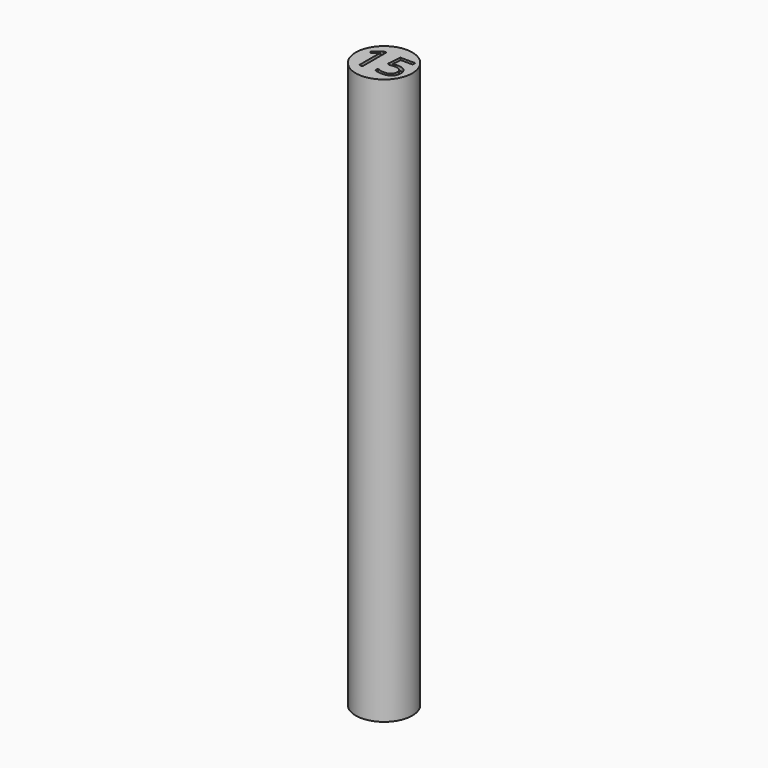
from build123d import *

# Parameters (mm, degrees)
F0_R         = 7.5
F1_DEPTH     = 150
F2_TEXT_SIZE = 11.1111111111
F3_DEPTH     = 1
F4_TEXT_SIZE = 11.1111111111
F5_DEPTH     = 1


# Not quite as in the source:
# - Text() gives the source's letters only with a copy of the font that has no kerning and outlines rounded to 1/6400 em; it was checked with that copy


with BuildPart() as f1:
    # F0 (on Top) → F1 (new body)
    with BuildSketch(Plane.XY):
        Circle(F0_R)
    extrude(amount=F1_DEPTH)

    # F2 (on face) → F3 (cut)
    with BuildSketch(Plane.XY.offset(150)):
        with Locations((-6.3932291667, -4)):
            Text('15', F2_TEXT_SIZE, font='Open Sans', text_align=(TextAlign.LEFT, TextAlign.BOTTOM))
    extrude(amount=-F3_DEPTH, mode=Mode.SUBTRACT)

    # F4 (on face) → F5 (cut)
    with BuildSketch(Plane(origin=(0, 0, 0), x_dir=(1, 0, 0), z_dir=(0, 0, -1))):
        with Locations((-6.3932291667, -4)):
            Text('15', F4_TEXT_SIZE, font='Open Sans', text_align=(TextAlign.LEFT, TextAlign.BOTTOM))
    extrude(amount=-F5_DEPTH, mode=Mode.SUBTRACT)


solid = f1.part
